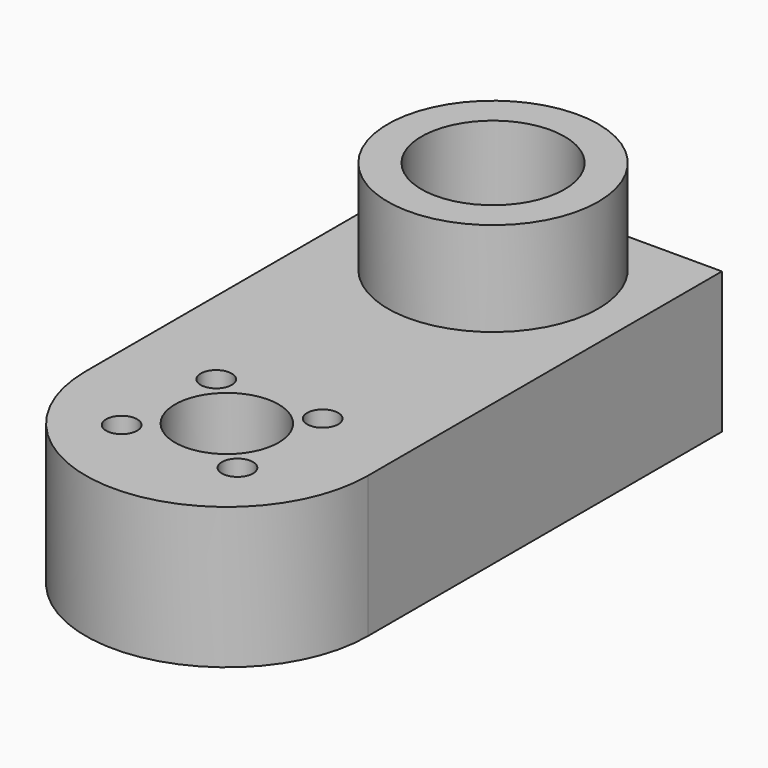
from build123d import *

# Parameters (mm, degrees)
F0_R     = 1.65
F0_R_2   = 5.5
F0_R_3   = 11.1803398875
F1_DEPTH = 15
F0_R_4   = 7.6
F2_DEPTH = 25


# Not quite as in the source:
# - a feature names something its author has since deleted; it is built from what else it names


with BuildPart() as f1:
    # F0 (on Top) → F1 (new body)
    with BuildSketch(Plane.XY):
        with BuildLine():
            Line((-19.2339122487, 8.4197289313), (-19.2339122487, 53.7750689313))
            Line((-19.2339122487, 53.7750689313), (-19.2339122487, 55.4197289313))
            Line((-19.2339122487, 55.4197289313), (-49.2339122487, 55.4197289313))
            Line((-49.2339122487, 55.4197289313), (-49.2339122487, 8.4197289313))
            ThreePointArc((-49.2339122487, 8.4197289313), (-34.2339122487, -6.5802710687), (-19.2339122487, 8.4197289313))
        make_face()
        with Locations((-40.8839122487, 2.7628746818)):
            Circle(F0_R, mode=Mode.SUBTRACT)
        with Locations((-39.8907664982, 14.0765831808)):
            Circle(F0_R, mode=Mode.SUBTRACT)
        with Locations((-34.2339122487, 8.4197289313)):
            Circle(F0_R_2, mode=Mode.SUBTRACT)
        with Locations((-28.5770579992, 2.7628746818)):
            Circle(F0_R, mode=Mode.SUBTRACT)
        with Locations((-28.5770579992, 14.0765831808)):
            Circle(F0_R, mode=Mode.SUBTRACT)
        with Locations((-34.2339122487, 43.7750689313)):
            Circle(F0_R_3, mode=Mode.SUBTRACT)
    extrude(amount=F1_DEPTH)

    # F0 (on Top) → F2 (join)
    with BuildSketch(Plane.XY):
        with Locations((-34.2339122487, 43.7750689313)):
            Circle(F0_R_3)
        with Locations((-34.2339122487, 43.7750689313)):
            Circle(F0_R_4, mode=Mode.SUBTRACT)
    extrude(amount=F2_DEPTH)


solid = f1.part
